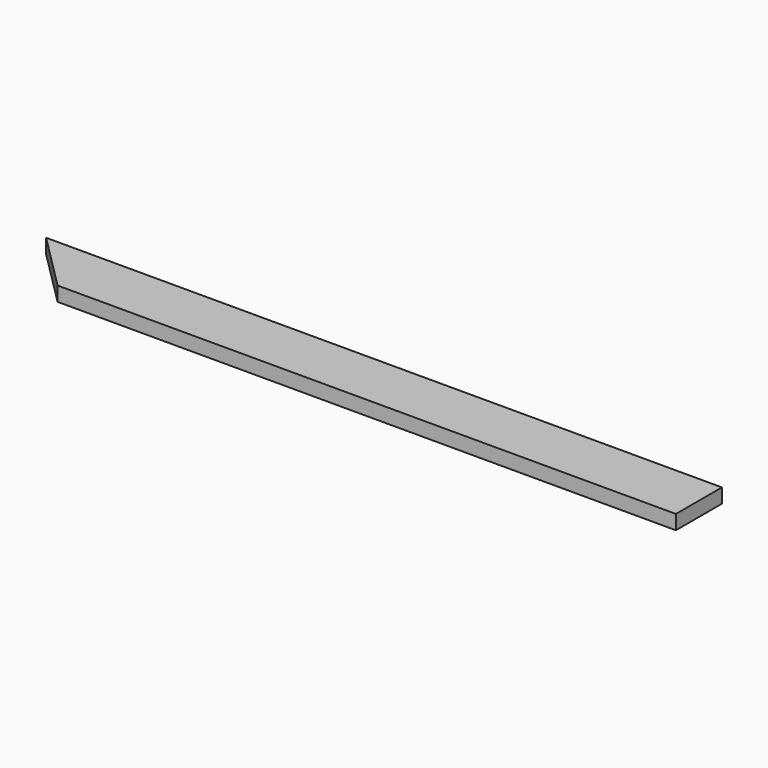
from build123d import *

# Parameters (mm, degrees)
F0_W     = 423
F0_H     = 36
F1_DEPTH = 9
F2_SIZE  = 35.99999


# Not quite as in the source:
# - a fillet or chamfer is up to 0.001 mm smaller than in the source, because OpenCascade refuses the exact size


with BuildPart() as f1:
    # F0 (on Top) → F1 (new body)
    with BuildSketch(Plane.XY):
        Rectangle(F0_W, F0_H)
    extrude(amount=F1_DEPTH)

    # F2 (size 36 in the source; OpenCascade refuses exactly that, so slightly less here)
    f2_edges = [f1.edges().sort_by_distance(p)[0] for p in [
        (-211.5, -18, 4.5),
    ]]
    chamfer(f2_edges, length=F2_SIZE)


solid = f1.part
